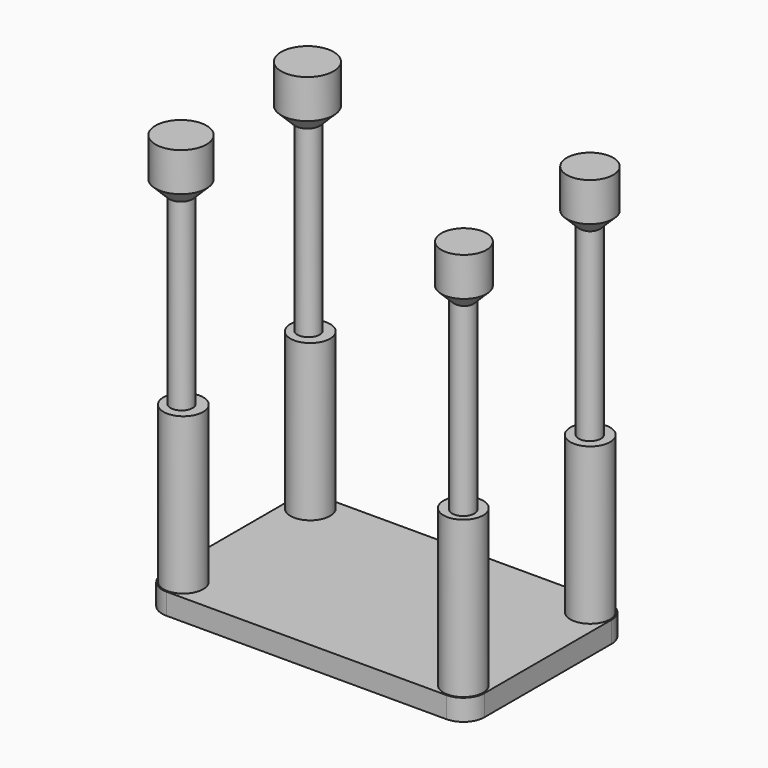
from build123d import *

# Parameters (mm, degrees)
F1_DEPTH     = 6.35
F2_R         = 5.9452870566
F3_DEPTH     = 46.736
F4_R         = 3.3233318127
F5_DEPTH     = 110.236
F7_START     = 108.204
F6_R         = 7.8492612618
F6_R_2       = 7.6458831821
F6_R_3       = 6.963642992
F6_R_4       = 6.7625316393
F7_DEPTH     = 15.748
F8_S9_R      = 3.3233318127
F8_T10_DEPTH = 11
F8_S15_R     = 3.3233318127
F8_T16_DEPTH = 12


# Not quite as in the source:
# - a fillet or chamfer that OpenCascade refuses, or shapes differently, is made with other operations: its cross-section is extruded or revolved along the edge and cut away or added


with BuildPart() as f1:
    # F0 (on Top) → F1 (new body)
    with BuildSketch(Plane.XY):
        with BuildLine():
            Line((17.025944097, 9.4035214942), (-66.794055903, 9.4035214942))
            ThreePointArc((-66.794055903, 9.4035214942), (-71.2841839635, 7.5436495547), (-73.144055903, 3.0535214942))
            Line((-73.144055903, 3.0535214942), (-73.144055903, -44.4444785058))
            ThreePointArc((-73.144055903, -44.4444785058), (-71.2841839635, -48.9346065664), (-66.794055903, -50.7944785058))
            Line((-66.794055903, -50.7944785058), (17.025944097, -50.7944785058))
            ThreePointArc((17.025944097, -50.7944785058), (21.5160721576, -48.9346065664), (23.375944097, -44.4444785058))
            Line((23.375944097, -44.4444785058), (23.375944097, 3.0535214942))
            ThreePointArc((23.375944097, 3.0535214942), (21.5160721576, 7.5436495547), (17.025944097, 9.4035214942))
        make_face()
    extrude(amount=F1_DEPTH)

    # F2 (on face) → F3 (join)
    with BuildSketch(Plane.XY.offset(6.35)):
        with Locations((-66.794055903, 3.0535214942)):
            Circle(F2_R)
        with Locations((17.025944097, 3.0535214942)):
            Circle(F2_R)
        with Locations((-66.794055903, -44.4444785058)):
            Circle(F2_R)
        with Locations((17.025944097, -44.4444785058)):
            Circle(F2_R)
    extrude(amount=F3_DEPTH)

    # F4 (on Top) → F5 (join)
    with BuildSketch(Plane.XY):
        with Locations((-67.3308223486, 3.0604917556)):
            Circle(F4_R)
        with Locations((16.9055722654, 3.0604917556)):
            Circle(F4_R)
        with Locations((-67.3308223486, -44.4500036538)):
            Circle(F4_R)
        with Locations((17.4885243177, -45.0329519808)):
            Circle(F4_R)
    extrude(amount=F5_DEPTH)

    # F6 (on Top) → F7 (join)
    with BuildSketch(Plane.XY.offset(F7_START)):
        with Locations((-67.5922632217, 2.9914693441)):
            Circle(F6_R)
        with Locations((-67.435964942, -44.5234365761)):
            Circle(F6_R_2)
        with Locations((17.121816054, 2.8351708315)):
            Circle(F6_R_3)
        with Locations((17.9033093154, -45.3049317002)):
            Circle(F6_R_4)
    extrude(amount=F7_DEPTH)

    # F8: chamfer of 4.1402 on 4 edges, made by hand

    # F8_s1 → F8_t2 (revolve, cut)
    with BuildSketch(Plane.XZ.offset(44.5234365761)):
        Polygon((-63.9302817599, 108.204), (-59.7900817599, 112.3442), (-59.7900817599, 108.204), align=None)
    revolve(axis=Axis((-67.435964942, -44.5234365761, 108.204), (0, 0, 1)), mode=Mode.SUBTRACT)

    # F8_s3 → F8_t4 (revolve, cut)
    with BuildSketch(Plane.XZ.offset(-2.9914693441)):
        Polygon((-63.8832019599, 108.204), (-59.7430019599, 112.3442), (-59.7430019599, 108.204), align=None)
    revolve(axis=Axis((-67.5922632217, 2.9914693441, 108.204), (0, 0, 1)), mode=Mode.SUBTRACT)


with BuildPart() as f8_tool6:
    # F8_s7 → F8_t8 (revolve)
    with BuildSketch(Plane.XZ.offset(45.3049317002)):
        Polygon((20.5256409548, 108.204), (24.6658409548, 112.3442), (24.6658409548, 108.204), align=None)
    revolve(axis=Axis((17.9033093154, -45.3049317002, 108.204), (0, 0, 1)))

    # F8_s9 → F8_t10 (cut, symmetric)
    with BuildSketch(Plane.XY.offset(110.3)):
        with Locations((17.4885243177, -45.0329519808)):
            Circle(F8_S9_R)
    extrude(amount=F8_T10_DEPTH, both=True, mode=Mode.SUBTRACT)


with BuildPart() as f1_1:
    add(f1.part)

    # F8_t5: cut F8_tool6
    add(f8_tool6.part, mode=Mode.SUBTRACT)


with BuildPart() as f8_tool12:
    # F8_s13 → F8_t14 (revolve)
    with BuildSketch(Plane.XZ.offset(-2.8351708315)):
        Polygon((19.945259046, 108.204), (24.085459046, 112.3442), (24.085459046, 108.204), align=None)
    revolve(axis=Axis((17.121816054, 2.8351708315, 108.204), (0, 0, 1)))

    # F8_s15 → F8_t16 (cut, symmetric)
    with BuildSketch(Plane.XY.offset(110.3)):
        with Locations((16.9055722654, 3.0604917556)):
            Circle(F8_S15_R)
    extrude(amount=F8_T16_DEPTH, both=True, mode=Mode.SUBTRACT)


with BuildPart() as f1_2:
    add(f1_1.part)

    # F8_t11: cut F8_tool12
    add(f8_tool12.part, mode=Mode.SUBTRACT)


solid = f1_2.part
